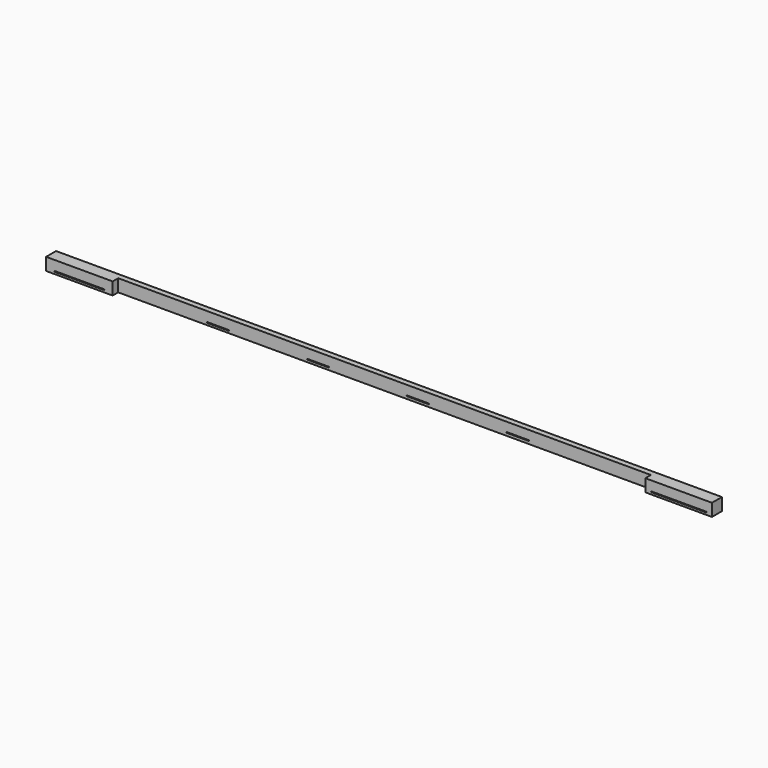
from build123d import *

# Parameters (mm, degrees)
F0_W      = 3048
F0_H      = 57.15
F2_DEPTH  = 57.15
F3_W      = 2438.4
F3_H      = 31.75
F4_DEPTH  = 57.15
F5_W      = 228.6
F5_H      = 3.429
F6_DEPTH  = 19.05
F7_W      = 254
F7_H      = 3.429
F8_DEPTH  = 19.05
F9_W      = 101.6
F9_H      = 3.429
F10_DEPTH = 19.05
F12_DEPTH = 9.525


# Not quite as in the source:
# - a variable given as a bare number and used for a length is read in inches; the dataset says mm whatever the document's units were


with BuildPart() as f2:
    # F0 (on Top) → F2 (new body)
    with BuildSketch(Plane.XY):
        with Locations((-4.8593655229, -305.1746997266)):
            Rectangle(F0_W, F0_H)
    extrude(amount=F2_DEPTH)

    # F3 (on face) → F4 (cut, through all)
    with BuildSketch(Plane.XY.offset(57.15)):
        with Locations((-4.8593655229, -317.8746997266)):
            Rectangle(F3_W, F3_H)
    extrude(amount=-F4_DEPTH, mode=Mode.SUBTRACT)

    # F5 (on face) → F6 (cut)
    with BuildSketch(Plane.XZ.offset(333.7496997266)):
        with Locations((-1376.4593655229, 11.2395)):
            Rectangle(F5_W, F5_H)
    extrude(amount=-F6_DEPTH, mode=Mode.SUBTRACT)

    # F7 (on face) → F8 (cut)
    with BuildSketch(Plane.XZ.offset(333.7496997266)):
        with Locations((1366.7406344771, 11.2395)):
            Rectangle(F7_W, F7_H)
    extrude(amount=-F8_DEPTH, mode=Mode.SUBTRACT)

    # F9 (on face) → F10 (cut)
    with BuildSketch(Plane.XZ.offset(301.9996997266)):
        with Locations((-766.8593655229, 11.2395)):
            Rectangle(F9_W, F9_H)
        with Locations((-309.6602423327, 12.1349072401)):
            Rectangle(F9_W, F9_H)
        with Locations((147.5388808575, 13.0303144803)):
            Rectangle(F9_W, F9_H)
        with Locations((604.7380040477, 13.9257217204)):
            Rectangle(F9_W, F9_H)
    extrude(amount=-F10_DEPTH, mode=Mode.SUBTRACT)

    # F11 (on face) → F12 (cut, through all)
    with BuildSketch(Plane.XY.offset(9.525)):
        with BuildLine():
            Line((-754.1593655229, -289.9346997266), (-766.8593655229, -289.9346997266))
            ThreePointArc((-766.8593655229, -289.9346997266), (-769.3993655229, -292.4746997266), (-766.8593655229, -295.0146997266))
            Line((-766.8593655229, -295.0146997266), (-754.1593655229, -295.0146997266))
            ThreePointArc((-754.1593655229, -295.0146997266), (-751.6193655229, -292.4746997266), (-754.1593655229, -289.9346997266))
        make_face()
    extrude(amount=-F12_DEPTH, mode=Mode.SUBTRACT)


solid = f2.part
